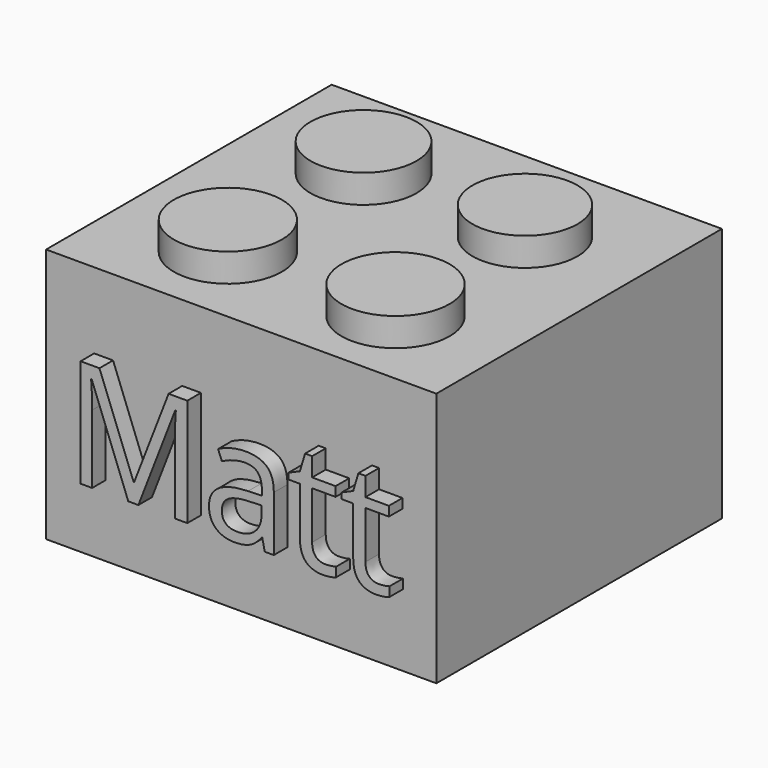
from build123d import *

# Parameters (mm, degrees)
F0_W         = 68.8704624772
F0_H         = 62.9953667521
F1_DEPTH     = 45
F2_R         = 9.3602645459
F2_R_2       = 9.2669038773
F2_R_3       = 9.5312181478
F2_R_4       = 9.5396708297
F3_DEPTH     = 5
F4_W         = 62.9999993835
F4_H         = 56.6999993753
F4_R         = 9.0962734323
F5_DEPTH     = 35
F6_TEXT_SIZE = 26.6477310409
F7_DEPTH     = 3


# Not quite as in the source:
# - Text() gives the source's letters only with a copy of the font that has no kerning and outlines rounded to 1/6400 em; it was checked with that copy


with BuildPart() as f1:
    # F0 (on Top) → F1 (new body)
    with BuildSketch(Plane.XY):
        with Locations((34.4352312386, 31.4976833761)):
            Rectangle(F0_W, F0_H)
    extrude(amount=F1_DEPTH)

    # F2 (on face) → F3 (join)
    with BuildSketch(Plane.XY.offset(45)):
        with Locations((20, 45.0294172647)):
            Circle(F2_R)
        with Locations((49.1847474056, 44.166109609)):
            Circle(F2_R_2)
        with Locations((20, 15.1013595694)):
            Circle(F2_R_3)
        with Locations((50.0480588049, 14.5258192604)):
            Circle(F2_R_4)
    extrude(amount=F3_DEPTH)

    # F4 (on face) → F5 (cut)
    with BuildSketch(Plane(origin=(0, 0, 0), x_dir=(1, 0, 0), z_dir=(0, 0, -1))):
        with Locations((34.5068172319, -31.5046381438)):
            Rectangle(F4_W, F4_H)
        with Locations((33.3613678813, -31.7910015583)):
            Circle(F4_R, mode=Mode.SUBTRACT)
    extrude(amount=-F5_DEPTH, mode=Mode.SUBTRACT)

    # F6 (on face) → F7 (join)
    with BuildSketch(Plane.XZ):
        with Locations((5.8704637922, 12.59536203)):
            Text('Matt', F6_TEXT_SIZE, font='Open Sans', text_align=(TextAlign.LEFT, TextAlign.BOTTOM))
    extrude(amount=F7_DEPTH)


solid = f1.part
